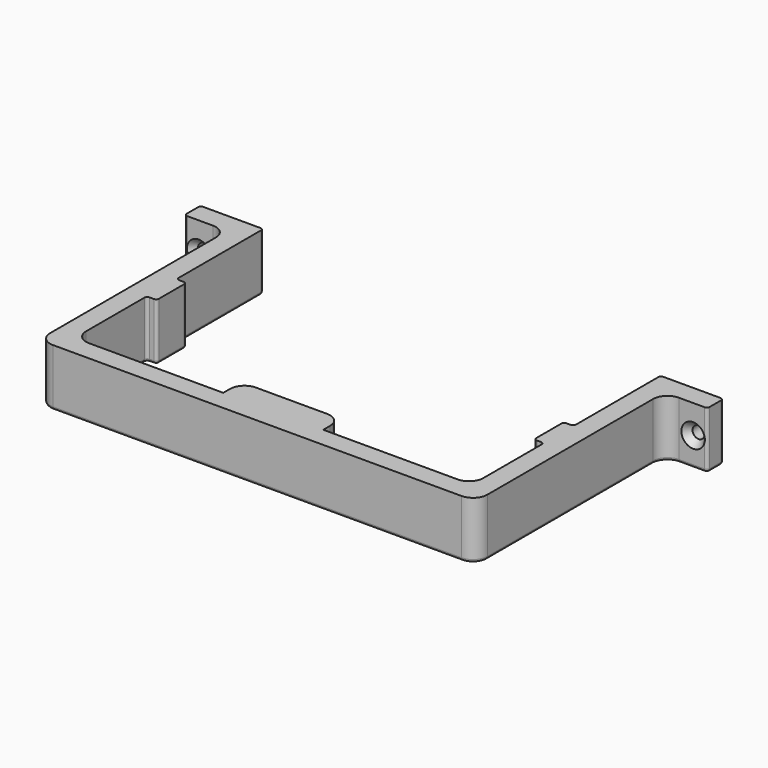
from build123d import *

# Parameters (mm, degrees)
F1_DEPTH             = 20
F4_D                 = 4.2
F4_CSINK_D           = 8.2
F4_CSINK_ANGLE       = 80
F4_ON_F2_D           = 4.2
F4_ON_F2_CSINK_D     = 8.2
F4_ON_F2_CSINK_ANGLE = 80
F5_T1_DEPTH          = 20
F5_T3_DEPTH          = 25
F6_R                 = 5
F7_R                 = 1


# Not quite as in the source:
# - a fillet or chamfer that OpenCascade refuses, or shapes differently, is made with other operations: its cross-section is extruded or revolved along the edge and cut away or added


with BuildPart() as f1:
    # F0 (on Top) → F1 (new body)
    with BuildSketch(Plane.XY):
        with BuildLine():
            Line((-74.0278660059, -17.2093475759), (-70.5278660059, -17.2093475759))
            Line((-70.5278660059, -17.2093475759), (-70.5278660059, -4.2093475759))
            Line((-70.5278660059, -4.2093475759), (-74.0278660059, -4.2093475759))
            Line((-74.0278660059, -4.2093475759), (-74.0278660059, 33.7906524241))
            Line((-74.0278660059, 33.7906524241), (-81.0278660059, 33.7906524241))
            Line((-81.0278660059, 33.7906524241), (-96.0278660059, 33.7906524241))
            Line((-96.0278660059, 33.7906524241), (-96.0278660059, 26.7906524241))
            Line((-96.0278660059, 26.7906524241), (-86.0278660059, 26.7906524241))
            ThreePointArc((-86.0278660059, 26.7906524241), (-82.4923321, 25.32618633), (-81.0278660059, 21.7906524241))
            Line((-81.0278660059, 21.7906524241), (-81.0278660059, -48.7093475759))
            Line((-81.0278660059, -48.7093475759), (-81.0278660059, -50.7093475759))
            ThreePointArc((-81.0278660059, -50.7093475759), (-79.5633999118, -54.2448814818), (-76.0278660059, -55.7093475759))
            Line((-76.0278660059, -55.7093475759), (-48.0278660059, -55.7093475759))
            Line((-48.0278660059, -55.7093475759), (-4.5278660059, -55.7093475759))
            Line((-4.5278660059, -55.7093475759), (38.9721339941, -55.7093475759))
            Line((38.9721339941, -55.7093475759), (66.9721339941, -55.7093475759))
            ThreePointArc((66.9721339941, -55.7093475759), (70.5076679, -54.2448814818), (71.9721339941, -50.7093475759))
            Line((71.9721339941, -50.7093475759), (71.9721339941, -48.7093475759))
            Line((71.9721339941, -48.7093475759), (71.9721339941, 21.7906524241))
            ThreePointArc((71.9721339941, 21.7906524241), (73.4366000882, 25.32618633), (76.9721339941, 26.7906524241))
            Line((76.9721339941, 26.7906524241), (86.9721339941, 26.7906524241))
            Line((86.9721339941, 26.7906524241), (86.9721339941, 33.7906524241))
            Line((86.9721339941, 33.7906524241), (71.9721339941, 33.7906524241))
            Line((71.9721339941, 33.7906524241), (64.9721339941, 33.7906524241))
            Line((64.9721339941, 33.7906524241), (64.9721339941, -4.2093475759))
            Line((64.9721339941, -4.2093475759), (61.4721339941, -4.2093475759))
            Line((61.4721339941, -4.2093475759), (61.4721339941, -17.2093475759))
            Line((61.4721339941, -17.2093475759), (64.9721339941, -17.2093475759))
            Line((64.9721339941, -17.2093475759), (64.9721339941, -48.7093475759))
            Line((64.9721339941, -48.7093475759), (12.9721339941, -48.7093475759))
            Line((12.9721339941, -48.7093475759), (12.9721339941, -45.7093475759))
            ThreePointArc((12.9721339941, -45.7093475759), (11.5076679, -42.17381367), (7.9721339941, -40.7093475759))
            Line((7.9721339941, -40.7093475759), (-4.5278660059, -40.7093475759))
            Line((-4.5278660059, -40.7093475759), (-17.0278660059, -40.7093475759))
            ThreePointArc((-17.0278660059, -40.7093475759), (-20.5633999118, -42.17381367), (-22.0278660059, -45.7093475759))
            Line((-22.0278660059, -45.7093475759), (-22.0278660059, -48.7093475759))
            Line((-22.0278660059, -48.7093475759), (-74.0278660059, -48.7093475759))
            Line((-74.0278660059, -48.7093475759), (-74.0278660059, -17.2093475759))
        make_face()
    extrude(amount=F1_DEPTH)

    # F4 (through all)
    with Locations(Plane.XZ.offset(-26.7906524241)):
        with Locations((81.9721339941, 10)):
            CounterSinkHole(F4_D / 2, F4_CSINK_D / 2, counter_sink_angle=F4_CSINK_ANGLE)

    # F4 on F2 (through all)
    with Locations(Plane.XZ.offset(-26.7906524241)):
        with Locations((-91.0278660059, 10)):
            CounterSinkHole(F4_ON_F2_D / 2, F4_ON_F2_CSINK_D / 2, counter_sink_angle=F4_ON_F2_CSINK_ANGLE)

    # F5: fillet of radius 1 on 14 edges, made by hand

    # F5_s2 → F5_t1 (join)
    with BuildSketch(Plane.XY):
        with BuildLine():
            ThreePointArc((-73.0278660059, -4.2093475759), (-73.7349727871, -3.9164543571), (-74.0278660059, -3.2093475759))
            Line((-74.0278660059, -3.2093475759), (-74.0278660059, -4.2093475759))
            Line((-74.0278660059, -4.2093475759), (-73.0278660059, -4.2093475759))
        make_face()
        with BuildLine():
            ThreePointArc((-74.0278660059, -18.2093475759), (-73.7349727871, -17.5022407947), (-73.0278660059, -17.2093475759))
            Line((-73.0278660059, -17.2093475759), (-74.0278660059, -17.2093475759))
            Line((-74.0278660059, -17.2093475759), (-74.0278660059, -18.2093475759))
        make_face()
        with BuildLine():
            ThreePointArc((64.9721339941, -18.2093475759), (64.6792407753, -17.5022407947), (63.9721339941, -17.2093475759))
            Line((63.9721339941, -17.2093475759), (64.9721339941, -17.2093475759))
            Line((64.9721339941, -17.2093475759), (64.9721339941, -18.2093475759))
        make_face()
        with BuildLine():
            ThreePointArc((64.9721339941, -3.2093475759), (64.6792407753, -3.9164543571), (63.9721339941, -4.2093475759))
            Line((63.9721339941, -4.2093475759), (64.9721339941, -4.2093475759))
            Line((64.9721339941, -4.2093475759), (64.9721339941, -3.2093475759))
        make_face()
    extrude(amount=F5_T1_DEPTH)

    # F5_s4 → F5_t3 (cut)
    with BuildSketch(Plane.XY.offset(-2.5)):
        with BuildLine():
            ThreePointArc((65.9721339941, 33.7906524241), (65.2650272129, 33.4977592053), (64.9721339941, 32.7906524241))
            Line((64.9721339941, 32.7906524241), (64.9721339941, 33.7906524241))
            Line((64.9721339941, 33.7906524241), (65.9721339941, 33.7906524241))
        make_face()
        with BuildLine():
            ThreePointArc((62.4721339941, -4.2093475759), (61.7650272129, -4.5022407947), (61.4721339941, -5.2093475759))
            Line((61.4721339941, -5.2093475759), (61.4721339941, -4.2093475759))
            Line((61.4721339941, -4.2093475759), (62.4721339941, -4.2093475759))
        make_face()
        with BuildLine():
            ThreePointArc((61.4721339941, -16.2093475759), (61.7650272129, -16.9164543571), (62.4721339941, -17.2093475759))
            Line((62.4721339941, -17.2093475759), (61.4721339941, -17.2093475759))
            Line((61.4721339941, -17.2093475759), (61.4721339941, -16.2093475759))
        make_face()
        with BuildLine():
            ThreePointArc((-71.5278660059, -17.2093475759), (-70.8207592247, -16.9164543571), (-70.5278660059, -16.2093475759))
            Line((-70.5278660059, -16.2093475759), (-70.5278660059, -17.2093475759))
            Line((-70.5278660059, -17.2093475759), (-71.5278660059, -17.2093475759))
        make_face()
        with BuildLine():
            ThreePointArc((-74.0278660059, 32.7906524241), (-74.3207592247, 33.4977592053), (-75.0278660059, 33.7906524241))
            Line((-75.0278660059, 33.7906524241), (-74.0278660059, 33.7906524241))
            Line((-74.0278660059, 33.7906524241), (-74.0278660059, 32.7906524241))
        make_face()
        with BuildLine():
            ThreePointArc((85.9721339941, 26.7906524241), (86.6792407753, 27.0835456429), (86.9721339941, 27.7906524241))
            Line((86.9721339941, 27.7906524241), (86.9721339941, 26.7906524241))
            Line((86.9721339941, 26.7906524241), (85.9721339941, 26.7906524241))
        make_face()
        with BuildLine():
            ThreePointArc((86.9721339941, 32.7906524241), (86.6792407753, 33.4977592053), (85.9721339941, 33.7906524241))
            Line((85.9721339941, 33.7906524241), (86.9721339941, 33.7906524241))
            Line((86.9721339941, 33.7906524241), (86.9721339941, 32.7906524241))
        make_face()
        with BuildLine():
            ThreePointArc((-70.5278660059, -5.2093475759), (-70.8207592247, -4.5022407947), (-71.5278660059, -4.2093475759))
            Line((-71.5278660059, -4.2093475759), (-70.5278660059, -4.2093475759))
            Line((-70.5278660059, -4.2093475759), (-70.5278660059, -5.2093475759))
        make_face()
        with BuildLine():
            ThreePointArc((-95.0278660059, 33.7906524241), (-95.7349727871, 33.4977592053), (-96.0278660059, 32.7906524241))
            Line((-96.0278660059, 32.7906524241), (-96.0278660059, 33.7906524241))
            Line((-96.0278660059, 33.7906524241), (-95.0278660059, 33.7906524241))
        make_face()
        with BuildLine():
            ThreePointArc((-96.0278660059, 27.7906524241), (-95.7349727871, 27.0835456429), (-95.0278660059, 26.7906524241))
            Line((-95.0278660059, 26.7906524241), (-96.0278660059, 26.7906524241))
            Line((-96.0278660059, 26.7906524241), (-96.0278660059, 27.7906524241))
        make_face()
    extrude(amount=F5_T3_DEPTH, mode=Mode.SUBTRACT)

    # F6
    f6_edges = [f1.edges().sort_by_distance(p)[0] for p in [
        (64.972134, -48.709348, 10),
        (-74.027866, -48.709348, 10),
    ]]
    fillet(f6_edges, radius=F6_R)

    # F7
    f7_edges = [f1.edges().sort_by_distance(p)[0] for p in [
        (-74.027866, -30.959348, 0),
        (-72.5634, -47.244881, 0),
        (-73.734973, -17.502241, 0),
        (-45.527866, -48.709348, 0),
        (-72.277866, -17.209348, 0),
        (-22.027866, -47.209348, 0),
        (-70.820759, -16.916454, 0),
        (-20.5634, -42.173814, 0),
        (-70.527866, -10.709348, 0),
        (-4.527866, -40.709348, 0),
        (-70.820759, -4.502241, 0),
        (11.507668, -42.173814, 0),
        (-72.277866, -4.209348, 0),
        (12.972134, -47.209348, 0),
        (-73.734973, -3.916454, 0),
        (36.472134, -48.709348, 0),
        (-74.027866, 14.790652, 0),
        (63.507668, -47.244881, 0),
        (-74.320759, 33.497759, 0),
        (64.972134, -30.959348, 0),
        (-85.027866, 33.790652, 0),
        (64.679241, -17.502241, 0),
        (-95.734973, 33.497759, 0),
        (63.222134, -17.209348, 0),
        (-96.027866, 30.290652, 0),
        (61.765027, -16.916454, 0),
        (-95.734973, 27.083546, 0),
        (61.472134, -10.709348, 0),
        (-90.527866, 26.790652, 0),
        (61.765027, -4.502241, 0),
        (-82.492332, 25.326186, 0),
        (63.222134, -4.209348, 0),
        (-81.027866, -14.459348, 0),
        (64.679241, -3.916454, 0),
        (-79.5634, -54.244881, 0),
        (64.972134, 14.790652, 0),
        (-4.527866, -55.709348, 0),
        (65.265027, 33.497759, 0),
        (70.507668, -54.244881, 0),
        (75.972134, 33.790652, 0),
        (71.972134, -14.459348, 0),
        (86.679241, 33.497759, 0),
        (73.4366, 25.326186, 0),
        (86.972134, 30.290652, 0),
        (81.472134, 26.790652, 0),
        (86.679241, 27.083546, 0),
    ]]
    fillet(f7_edges, radius=F7_R)


solid = f1.part
